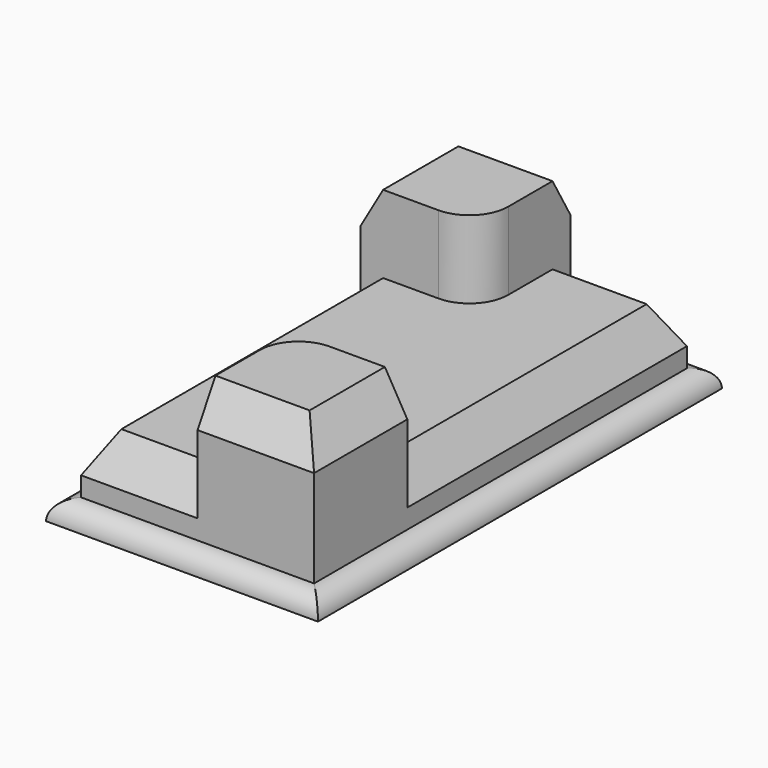
from build123d import *

# Parameters (mm, degrees)
F0_W     = 88.9
F0_H     = 165.1
F1_DEPTH = 6.35
F2_DEPTH = 25.4
F3_DEPTH = 50.8
F4_SIZE2 = 12.7
F4_SIZE  = 7.3323484187
F5_R     = 6.34999
F6_SIZE2 = 12.7
F6_SIZE  = 7.3323484187
F7_SIZE2 = 12.7
F7_SIZE  = 7.3323484187


# Not quite as in the source:
# - a fillet or chamfer is up to 0.001 mm smaller than in the source, because OpenCascade refuses the exact size


with BuildPart() as f1:
    # F0 (on Top) → F1 (new body)
    with BuildSketch(Plane.XY):
        Rectangle(F0_W, F0_H)
        Polygon((-38.1, 38.1), (-38.1, 76.2), (0, 76.2), (38.1, 76.2), (38.1, -38.1), (38.1, -76.2), (0, -76.2), (-38.1, -76.2), align=None, mode=Mode.SUBTRACT)
    extrude(amount=F1_DEPTH)

    # F0 (on Top) → F2 (join)
    with BuildSketch(Plane.XY):
        with BuildLine():
            Line((38.1, 76.2), (0, 76.2))
            Line((0, 76.2), (0, 50.8))
            ThreePointArc((0, 50.8), (-3.7197438789, 41.8197438789), (-12.7, 38.1))
            Line((-12.7, 38.1), (-38.1, 38.1))
            Line((-38.1, 38.1), (-38.1, -76.2))
            Line((-38.1, -76.2), (0, -76.2))
            Line((0, -76.2), (0, -50.8))
            ThreePointArc((0, -50.8), (3.7197438789, -41.8197438789), (12.7, -38.1))
            Line((12.7, -38.1), (38.1, -38.1))
            Line((38.1, -38.1), (38.1, 76.2))
        make_face()
    extrude(amount=F2_DEPTH)

    # F0 (on Top) → F3 (join)
    with BuildSketch(Plane.XY):
        with BuildLine():
            Line((0, 76.2), (-38.1, 76.2))
            Line((-38.1, 76.2), (-38.1, 38.1))
            Line((-38.1, 38.1), (-12.7, 38.1))
            ThreePointArc((-12.7, 38.1), (-3.7197438789, 41.8197438789), (0, 50.8))
            Line((0, 50.8), (0, 76.2))
        make_face()
        with BuildLine():
            Line((38.1, -76.2), (38.1, -38.1))
            Line((38.1, -38.1), (12.7, -38.1))
            ThreePointArc((12.7, -38.1), (3.7197438789, -41.8197438789), (0, -50.8))
            Line((0, -50.8), (0, -76.2))
            Line((0, -76.2), (38.1, -76.2))
        make_face()
    extrude(amount=F3_DEPTH)

    # F4
    f4_edges = [f1.edges().sort_by_distance(p)[0] for p in [
        (38.1, 19.05, 25.4),
        (-19.05, -76.2, 25.4),
        (-38.1, -19.05, 25.4),
        (19.05, 76.2, 25.4),
    ]]
    f4_side = f1.faces().sort_by_distance((0, 0, 25.4))[0]
    chamfer(f4_edges, length=F4_SIZE, length2=F4_SIZE2, reference=f4_side)

    # F5 (radius 6.35 in the source; OpenCascade refuses exactly that, so slightly less here)
    f5_edges = [f1.edges().sort_by_distance(p)[0] for p in [
        (0, 82.55, 6.35),
        (-44.45, 0, 6.35),
        (44.45, 0, 6.35),
        (0, -82.55, 6.35),
    ]]
    fillet(f5_edges, radius=F5_R)

    # F6
    f6_edges = [f1.edges().sort_by_distance(p)[0] for p in [
        (19.05, -76.2, 50.8),
        (38.1, -57.15, 50.8),
    ]]
    f6_side = f1.faces().sort_by_distance((19.446042, -57.546042, 50.8))[0]
    chamfer(f6_edges, length=F6_SIZE, length2=F6_SIZE2, reference=f6_side)

    # F7
    f7_edges = [f1.edges().sort_by_distance(p)[0] for p in [
        (-19.05, 76.2, 50.8),
        (-38.1, 57.15, 50.8),
    ]]
    f7_side = f1.faces().sort_by_distance((-19.446042, 57.546042, 50.8))[0]
    chamfer(f7_edges, length=F7_SIZE, length2=F7_SIZE2, reference=f7_side)


solid = f1.part
